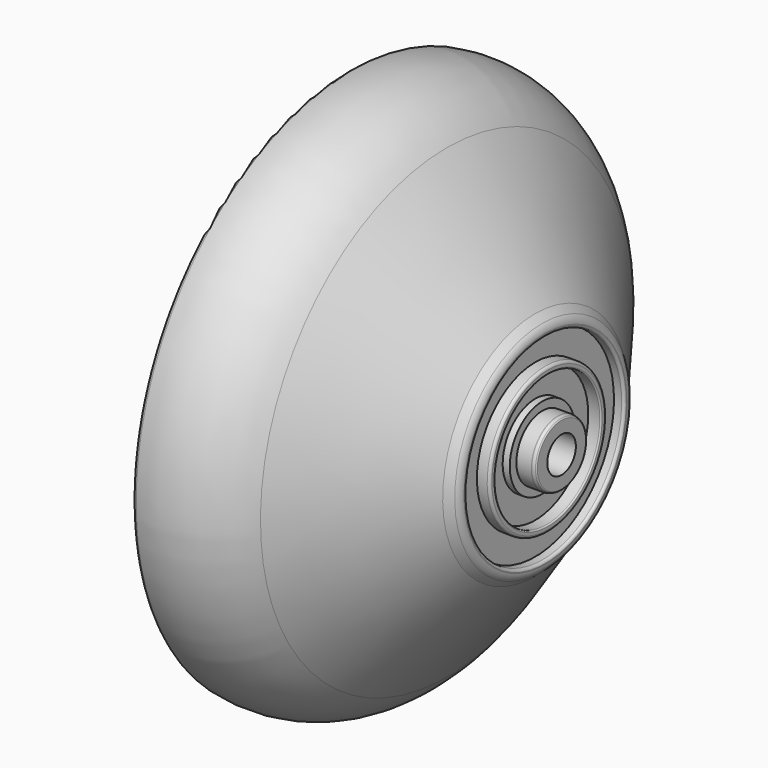
from build123d import *


# Not quite as in the source:
# - ends of sketch curves that miss each other by under 0.0002 mm in the source are joined


with BuildPart() as f1:
    # F0 (on Front) → F1 (revolve)
    with BuildSketch(Plane.XZ):
        with BuildLine():
            ThreePointArc((2.6699981334, 9.9816318545), (2.5858836167, 10.3828227138), (2.3477073858, 10.7164414191))
            Line((2.3477073858, 10.7164414191), (1.6664407013, 11.3436680393))
            Line((1.6664407013, 11.3436680393), (-6.9871413476, 22.8526270762))
            ThreePointArc((-6.9871413476, 22.8526270762), (-11.1053040379, 25.9865847738), (-16.2548080503, 26.4999688597))
            ThreePointArc((-16.2548080503, 26.4999688597), (-16.7414077187, 25.7816474852), (-16.1563307047, 25.1409839839))
            ThreePointArc((-16.1563307047, 25.1409839839), (-14.1032938688, 22.09460651), (-13.1370675801, 18.5503459776))
            ThreePointArc((-13.1370675801, 18.5503459776), (-12.780163443, 17.8472749816), (-12.044202136, 17.5643432885))
            Line((-12.044202136, 17.5643432885), (-6.0741969575, 17.5643432885))
            ThreePointArc((-6.0741969575, 17.5643432885), (-5.3287105343, 17.4945370263), (-4.7319698321, 17.0422943307))
            Line((-4.7319698321, 17.0422943307), (-0.2304927586, 11.0554885257))
            ThreePointArc((-0.2304927586, 11.0554885257), (0.0988031231, 10.4283951413), (0.2124717155, 9.7292804572))
            Line((0.2124717155, 9.7292804572), (0.2124717155, 4.0234341655))
            ThreePointArc((0.2124717155, 4.0234341655), (0.0523024795, 3.124834336), (-0.4084772998, 2.3369143954))
            ThreePointArc((-0.4084772998, 2.3369143954), (-1.2026479798, 1.2699423116), (-1.5981009122, 0))
            Line((-1.5981009122, 0), (0, 0))
            Line((0, 0), (1.054421, 1.754851))
            Line((1.054421, 1.754851), (4.24833, 1.754851))
            Line((4.24833, 1.754851), (4.24833, 2.965108))
            ThreePointArc((4.24833, 2.965108), (4.2243561549, 3.0393632641), (4.1614868664, 3.085580599))
            Line((4.1614868664, 3.085580599), (3.879268, 3.179662))
            ThreePointArc((3.879268, 3.179662), (3.8594525644, 3.1845473579), (3.83911, 3.18619))
            Line((3.83911, 3.18619), (2.36708, 3.18619))
            Line((2.36708, 3.18619), (2.36708, 3.998))
            Line((2.36708, 3.998), (1.672421, 3.998))
            Line((1.672421, 3.998), (1.672421, 6.492))
            Line((1.672421, 6.492), (2.801421, 6.492))
            ThreePointArc((2.801421, 6.492), (2.8912235612, 6.5291974388), (2.928421, 6.619))
            Line((2.928421, 6.619), (2.928421, 6.896))
            ThreePointArc((2.928421, 6.896), (2.8540261224, 7.0756051224), (2.674421, 7.15))
            Line((2.674421, 7.15), (1.668421, 7.15))
            Line((1.668421, 7.15), (1.668421, 7.150491))
            Line((1.668421, 7.150491), (1.668421, 9.65))
            Line((1.668421, 9.65), (1.668421, 9.65036))
            Line((1.668421, 9.65036), (2.419171, 9.651342))
            ThreePointArc((2.419171, 9.651342), (2.5987761224, 9.7257368776), (2.673171, 9.905342))
            Line((2.673171, 9.905342), (2.6699981334, 9.9816318545))
        make_face()
    revolve(axis=Axis((-0.7990504561, 0, 0), (-1, 0, 0)))


solid = f1.part
